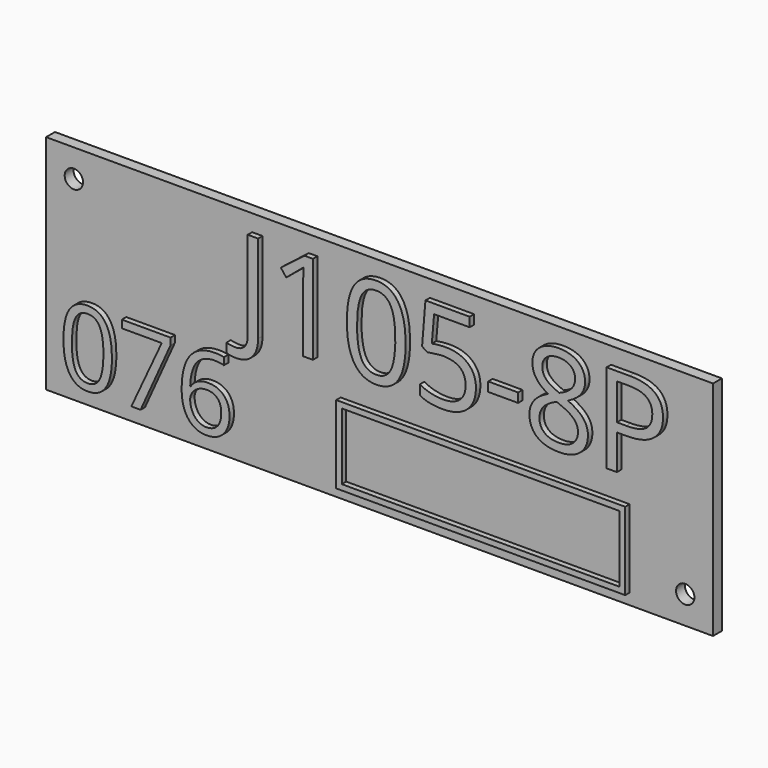
from build123d import *

# Parameters (mm, degrees)
F0_W         = 120
F0_H         = 40
F1_DEPTH     = 2
F3_D         = 3.3
F4_TEXT_SIZE = 22.4128874103
F5_DEPTH     = 1
F6_TEXT_SIZE = 18.4837545126
F7_DEPTH     = 1
F8_W         = 52
F8_H         = 14
F8_W_2       = 49.99999962
F8_H_2       = 11.99999962
F9_DEPTH     = 1


# Not quite as in the source:
# - Text() gives the source's letters only with a copy of the font that has no kerning and outlines rounded to 1/6400 em; it was checked with that copy


with BuildPart() as f1:
    # F0 (on Front) → F1 (new body)
    with BuildSketch(Plane.XZ):
        Rectangle(F0_W, F0_H)
    extrude(amount=F1_DEPTH)

    # F3 (through all)
    with Locations(Plane.XZ.offset(2)):
        with Locations((-55, 15), (55, -15)):
            Hole(F3_D / 2)

    # F4 (on face) → F5 (join)
    with BuildSketch(Plane.XZ.offset(2)):
        with Locations((-25, 1)):
            Text('J105-8P', F4_TEXT_SIZE, font='Open Sans', text_align=(TextAlign.LEFT, TextAlign.BOTTOM))
    extrude(amount=F5_DEPTH)

    # F6 (on face) → F7 (join)
    with BuildSketch(Plane.XZ.offset(2)):
        with Locations((-57, -17)):
            Text('076', F6_TEXT_SIZE, font='Open Sans', text_align=(TextAlign.LEFT, TextAlign.BOTTOM))
    extrude(amount=F7_DEPTH)

    # F8 (on face) → F9 (join)
    with BuildSketch(Plane.XZ.offset(2)):
        with Locations((19, -11)):
            Rectangle(F8_W, F8_H)
        with Locations((19, -11)):
            Rectangle(F8_W_2, F8_H_2, mode=Mode.SUBTRACT)
    extrude(amount=F9_DEPTH)


solid = f1.part
